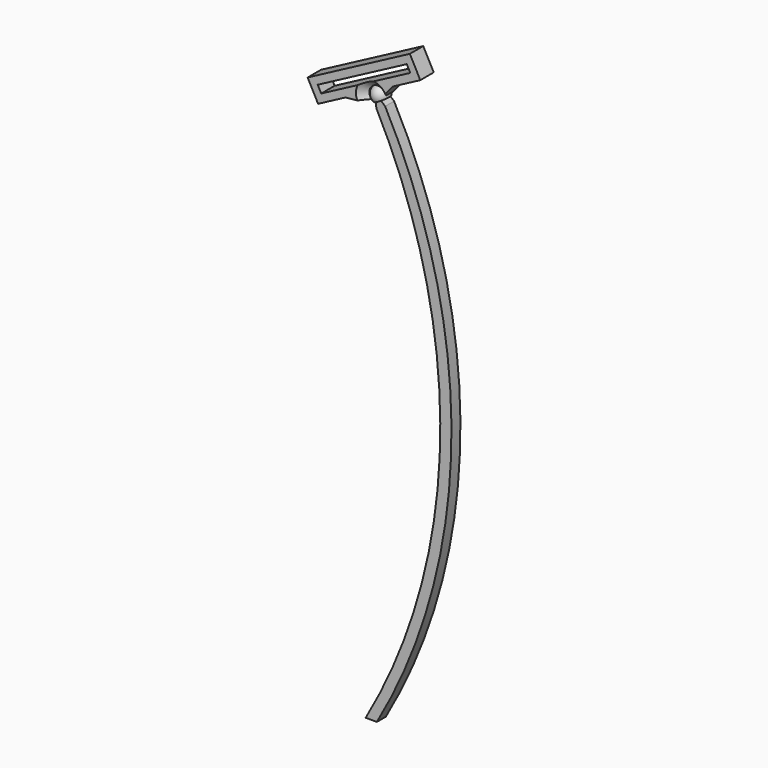
from build123d import *

# Parameters (mm, degrees)
F1_DEPTH      = 1.5
F6_DEPTH      = 2
F6_DEPTH_BACK = 3
F8_W          = 33.8980406523
F8_H          = 26.2241512537
F9_DEPTH      = 4
F10_T2_ANGLE  = 359.64


# Not quite as in the source:
# - a fillet or chamfer that OpenCascade refuses, or shapes differently, is made with other operations: its cross-section is extruded or revolved along the edge and cut away or added


with BuildPart() as f1:
    # F0 (on Front) → F1 (new body, symmetric)
    with BuildSketch(Plane.XZ):
        with BuildLine():
            ThreePointArc((2.874675002, 69.7547661407), (19.9703072521, -2.9906619086), (0, -75))
            Line((0, -75), (3, -75))
            ThreePointArc((3, -75), (22.9826005439, -2.2893849442), (5.2192689269, 70.9950057277))
            Line((5.2192689269, 70.9950057277), (3.9680614468, 72.0683399281))
            Line((3.9680614468, 72.0683399281), (3.9560562747, 72.0786384293))
            Line((3.9560562747, 72.0786384293), (2.6897316802, 71.4087800477))
            Line((2.6897316802, 71.4087800477), (2.874675002, 69.7547661407))
        make_face()
    extrude(amount=F1_DEPTH, both=True)

    # F2 (on Front) → F11 (revolve)
    with BuildSketch(Plane.XZ):
        with BuildLine():
            Line((3.4283745063, 71.5443050188), (2.259403264, 73.7541706787))
            ThreePointArc((2.259403264, 73.7541706787), (1.7389560552, 72.0647522276), (3.4283745063, 71.5443050188))
        make_face()
    revolve(axis=Axis((2.3768325607, 0, 73.5321780745), (-0.4675884969, 0, 0.8839462639)))


with BuildPart() as f4:
    # F3 (on Front) → F4 (revolve)
    with BuildSketch(Plane.XZ):
        with BuildLine():
            ThreePointArc((2.0443154021, 71.6242099246), (1.5489133531, 72.763423537), (2.2360238391, 73.7983679919))
            Line((2.2360238391, 73.7983679919), (1.7684353422, 74.6823142558))
            ThreePointArc((1.7684353422, 74.6823142558), (0.5450086387, 72.7209986501), (1.6437255478, 70.6871960643))
            Line((1.6437255478, 70.6871960643), (2.0443154021, 71.6242099246))
        make_face()
    revolve(axis=Axis((2.532587825, 0, 73.2377326703), (-0.4675884969, 0, 0.8839462639)))

    # F5 (on Front) → F6 (join, two sides)
    with BuildSketch(Plane.XZ) as f6_sk:
        with BuildLine():
            Line((-14.3645751176, 72.0319375121), (-11.559044136, 66.7282599284))
            Line((-11.559044136, 66.7282599284), (-4.2218675739, 70.6094679841))
            Line((-4.2218675739, 70.6094679841), (1.1471386437, 71.1712600625))
            ThreePointArc((1.1471386437, 71.1712600625), (1.7922159684, 74.637358497), (5.0204523013, 73.2201593963))
            Line((5.0204523013, 73.2201593963), (8.506113484, 77.3422952775))
            Line((8.506113484, 77.3422952775), (15.8432900462, 81.2235033332))
            Line((15.8432900462, 81.2235033332), (13.0377590646, 86.5271809169))
            Line((13.0377590646, 86.5271809169), (-14.3645751176, 72.0319375121))
        make_face()
        Polygon((-10.726328602, 69.4313294501), (-11.6615055959, 71.199221978), (12.2050435306, 83.8241113951), (13.1402205245, 82.0562188673), align=None, mode=Mode.SUBTRACT)
    extrude(amount=-F6_DEPTH)
    extrude(f6_sk.sketch, amount=F6_DEPTH_BACK)

    # F8 (on offset) → F9 (cut)
    with BuildSketch(Plane.XZ.offset(-1.5)):
        with Locations((0.1696329564, 77.5720775127)):
            Rectangle(F8_W, F8_H)
    extrude(amount=-F9_DEPTH, mode=Mode.SUBTRACT)

    # F10: chamfer of 2 on 1 edges, made by hand

    # F10_s1 → F10_t2 (revolve, cut)
    with BuildSketch(Plane(origin=(32.1280601549, 0, 16.8660881044), x_dir=(0, 1, 0), z_dir=(0.885410872, 0, 0.464809195))):
        Polygon((-1, 60.7517013138), (-3, 58.7517013138), (-3, 60.7517013138), align=None)
    revolve(axis=Axis((2.8442900865, -3, 72.6484794032), (0, 1, 0)), revolution_arc=F10_T2_ANGLE, mode=Mode.SUBTRACT)


solid = Compound([f1.part, f4.part])
